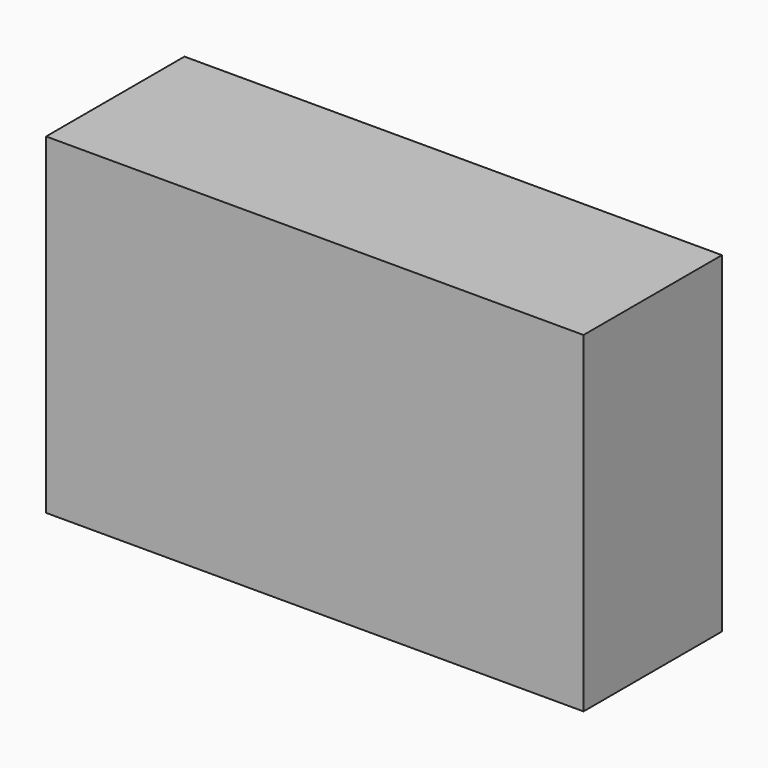
from build123d import *

# Parameters (mm, degrees)
F0_W     = 78.9205972105
F0_H     = 48.6620664597
F1_DEPTH = 25.4


# Not quite as in the source:
# - a feature of the source that left no trace in its solid (it failed there, or was rolled back) is left out


with BuildPart() as f1:
    # F0 (on Front) → F1 (new body)
    with BuildSketch(Plane.XZ):
        with Locations((13.4761175141, -0.5565732718)):
            Rectangle(F0_W, F0_H)
    extrude(amount=F1_DEPTH)


solid = f1.part
